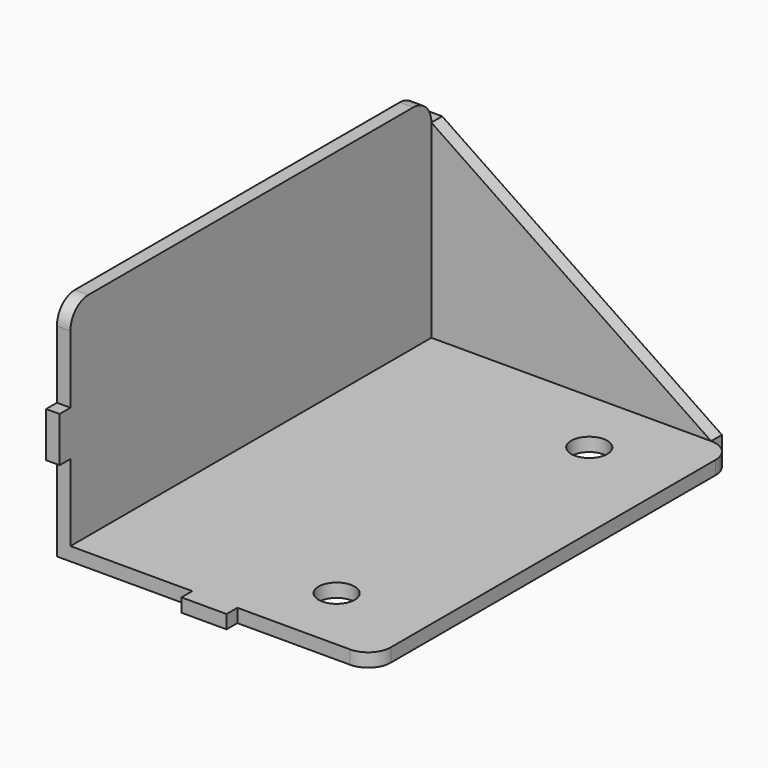
from build123d import *

# Parameters (mm, degrees)
F1_DEPTH = 100
F2_R     = 4
F3_DEPTH = 25
F5_DEPTH = 3
F7_R     = 5
F8_W     = 3
F8_H     = 15
F9_DEPTH = 3


# Not quite as in the source:
# - a pattern or mirror of a feature is missing from the dataset's text; its kind, count and spacing are read off the source's solid


with BuildPart() as f1:
    # F0 (on Front) → F1 (new body)
    with BuildSketch(Plane.XZ):
        Polygon((0, 50), (0, 0), (70, 0), (70, 3), (3, 3), (3, 50), align=None)
    extrude(amount=-F1_DEPTH)

    # F2 (on face) → F3 (cut)
    with BuildSketch(Plane.XY.offset(3)):
        with Locations((50, 85)):
            Circle(F2_R)
        with Locations((50, 15)):
            Circle(F2_R)
    extrude(amount=-F3_DEPTH, mode=Mode.SUBTRACT)

    # F4 (on face) → F5 (join)
    with BuildSketch(Plane(origin=(0, 100, 0), x_dir=(-1, 0, 0), z_dir=(0, 1, 0))):
        Polygon((-3, 20), (0, 20), (0, 25), (0, 30), (-3, 30), align=None)
        Polygon((-35, 0), (-30, 0), (-30, 3), (-40, 3), (-40, 0), align=None)
    f5 = extrude(amount=F5_DEPTH)

    # F5_copies: F5 across plane
    add(f5.mirror(Plane(origin=(0, 50, 0), x_dir=(0, 0, -1), z_dir=(0, -1, 0))))

    # F7
    f7_edges = [f1.edges().sort_by_distance(p)[0] for p in [
        (1.5, 100, 50),
        (1.5, 0, 50),
        (70, 100, 1.5),
        (70, 0, 1.5),
    ]]
    fillet(f7_edges, radius=F7_R)


with BuildPart() as f9:
    # F8 (on face) → F9 (new body)
    with BuildSketch(Plane(origin=(0, 100, 0), x_dir=(-1, 0, 0), z_dir=(0, 1, 0))):
        Polygon((-3, 20), (-3, 30), (-3, 45), (-65, 3), (-65, 0), (-40, 0), (-40, 3), (-30, 3), (-3, 3), align=None)
        Polygon((0, 20), (-3, 20), (-3, 3), (-30, 3), (-30, 0), (0, 0), align=None)
        with Locations((-1.5, 37.5)):
            Rectangle(F8_W, F8_H)
    extrude(amount=F9_DEPTH)


solid = Compound([f1.part, f9.part])
